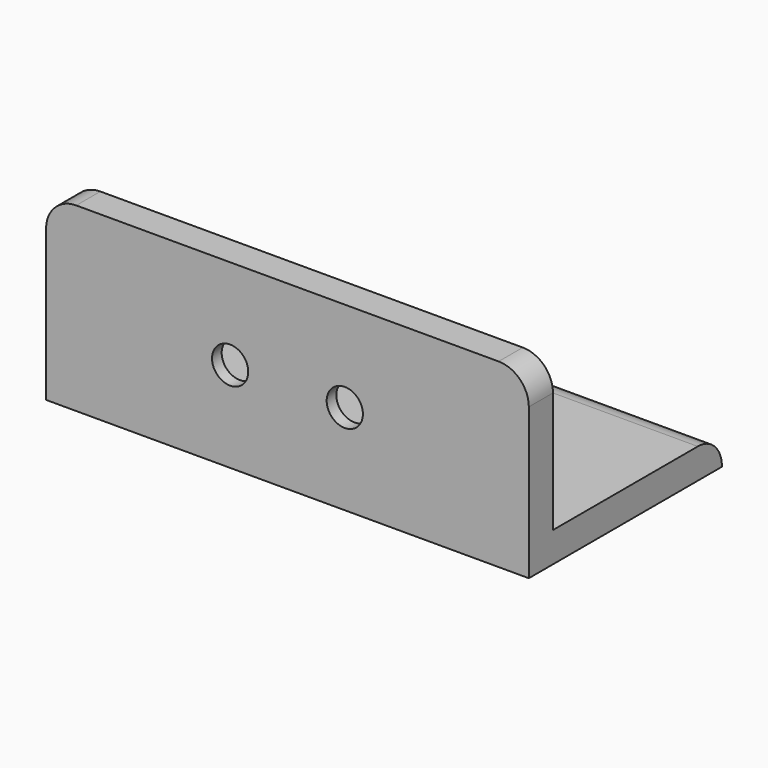
from build123d import *

# Parameters (mm, degrees)
F0_W     = 80
F0_H     = 40
F1_DEPTH = 5
F2_W     = 80
F2_H     = 25
F2_R     = 3
F3_DEPTH = 5
F4_R     = 4.99999
F5_R     = 3
F6_DEPTH = 3


# Not quite as in the source:
# - a fillet or chamfer is up to 0.001 mm smaller than in the source, because OpenCascade refuses the exact size


with BuildPart() as f1:
    # F0 (on Top) → F1 (new body)
    with BuildSketch(Plane.XY):
        with Locations((-1.6386443377, -15.6908366084)):
            Rectangle(F0_W, F0_H)
    extrude(amount=-F1_DEPTH)

    # F2 (on face) → F3 (join)
    with BuildSketch(Plane.XZ.offset(35.6908366084)):
        with Locations((-1.6386443377, 12.5)):
            Rectangle(F2_W, F2_H)
        with Locations((-11.1386443377, 10)):
            Circle(F2_R, mode=Mode.SUBTRACT)
        with Locations((7.8613556623, 10)):
            Circle(F2_R, mode=Mode.SUBTRACT)
    extrude(amount=-F3_DEPTH)

    # F4 (radius 5 in the source; OpenCascade refuses exactly that, so slightly less here)
    f4_edges = [f1.edges().sort_by_distance(p)[0] for p in [
        (-41.638644, -33.190837, 25),
        (38.361356, -33.190837, 25),
        (-1.638644, 4.309163, 0),
    ]]
    fillet(f4_edges, radius=F4_R)

    # F5 (on face) → F6 (cut)
    with BuildSketch(Plane(origin=(0, -30.6908366084, 0), x_dir=(-1, 0, 0), z_dir=(0, 1, 0))):
        with BuildLine():
            ThreePointArc((-7.8613556623, 1.5), (-1.8509480223, 3.9895923599), (0.6386443377, 10))
            ThreePointArc((0.6386443377, 10), (-1.8509480223, 16.0104076401), (-7.8613556623, 18.5))
            ThreePointArc((-7.8613556623, 18.5), (-16.3613556623, 10), (-7.8613556623, 1.5))
        make_face()
        with Locations((-7.8613556623, 10)):
            Circle(F5_R, mode=Mode.SUBTRACT)
        with BuildLine():
            ThreePointArc((-7.8613556623, 18.5), (-1.8509480223, 16.0104076401), (0.6386443377, 10))
            ThreePointArc((0.6386443377, 10), (-1.8509480223, 3.9895923599), (-7.8613556623, 1.5))
            Line((-7.8613556623, 1.5), (11.1386443377, 1.5))
            ThreePointArc((11.1386443377, 1.5), (2.6386443377, 10), (11.1386443377, 18.5))
            Line((11.1386443377, 18.5), (-7.8613556623, 18.5))
        make_face()
        with BuildLine():
            ThreePointArc((19.6386443377, 10), (17.1490519777, 16.0104076401), (11.1386443377, 18.5))
            ThreePointArc((11.1386443377, 18.5), (2.6386443377, 10), (11.1386443377, 1.5))
            ThreePointArc((11.1386443377, 1.5), (17.1490519777, 3.9895923599), (19.6386443377, 10))
        make_face()
        with Locations((11.1386443377, 10)):
            Circle(F5_R, mode=Mode.SUBTRACT)
        with Locations((11.1386443377, 10)):
            Circle(F5_R)
        with Locations((-7.8613556623, 10)):
            Circle(F5_R)
    extrude(amount=-F6_DEPTH, mode=Mode.SUBTRACT)


solid = f1.part
